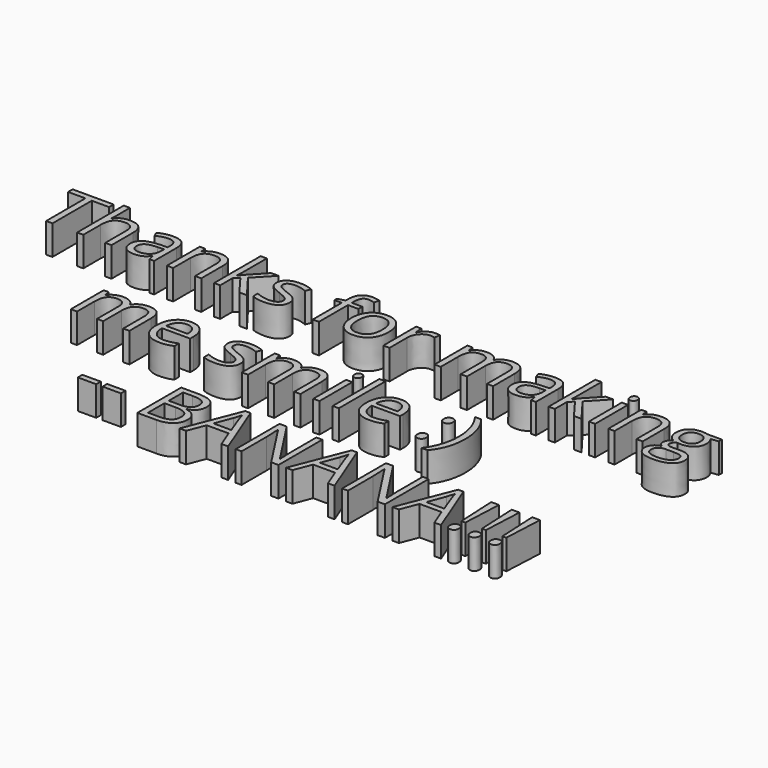
from build123d import *

# Parameters (mm, degrees)
F0_TEXT_SIZE = 5.18657254
F1_DEPTH     = 2


# Not quite as in the source:
# - Text() gives the source's letters only with a copy of the font that has no kerning and outlines rounded to 1/6400 em; it was checked with that copy


with BuildPart() as f1:
    # F0 (on Top) → F1 (new body)
    with BuildSketch(Plane.XY):
        with Locations((-22.5, 3.4780358705)):
            Text('Thanks for making', F0_TEXT_SIZE, font='Open Sans', text_align=(TextAlign.LEFT, TextAlign.BOTTOM))
        with Locations((-14.4138092494, -3.5757027838)):
            Text('me smile :)', F0_TEXT_SIZE, font='Open Sans', text_align=(TextAlign.LEFT, TextAlign.BOTTOM))
        with Locations((-9.0230154156, -10.6294414382)):
            Text('-- BANANA!!!', F0_TEXT_SIZE, font='Open Sans', text_align=(TextAlign.LEFT, TextAlign.BOTTOM))
    extrude(amount=F1_DEPTH)


solid = f1.part
